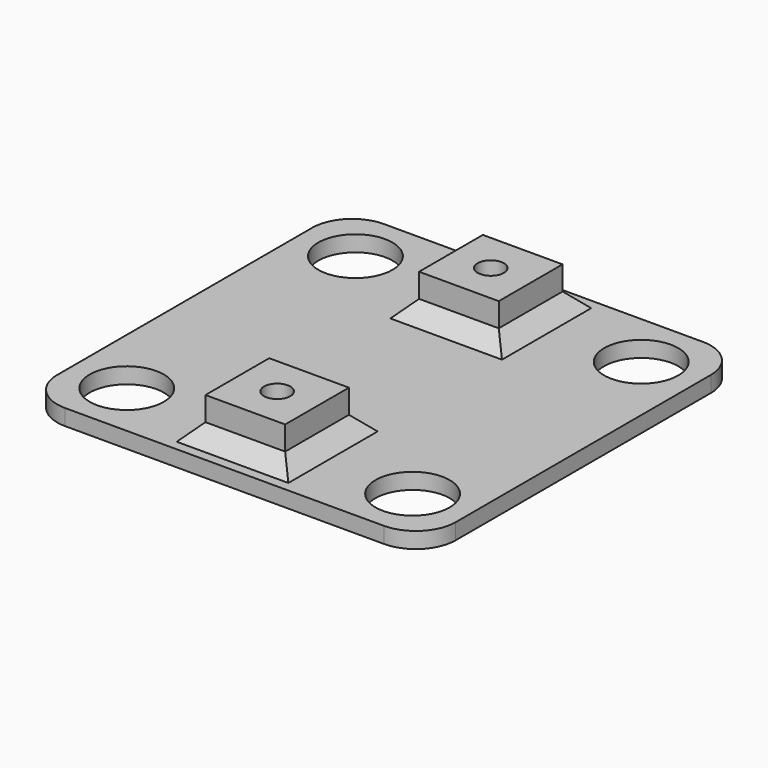
from build123d import *

# Parameters (mm, degrees)
F0_W     = 10
F0_H     = 10
F0_R     = 1.65
F1_DEPTH = 7
F0_R_2   = 4.65
F2_DEPTH = 2
F3_SIZE  = 2


with BuildPart() as f1:
    # F0 (on Top) → F1 (new body)
    with BuildSketch(Plane.XY):
        with Locations((25, -41.75)):
            Rectangle(F0_W, F0_H)
        with Locations((25, -41.75)):
            Circle(F0_R, mode=Mode.SUBTRACT)
    extrude(amount=F1_DEPTH)



with BuildPart() as f1b:
    # F0 (on Top) → F1, piece 2 (new body)
    with BuildSketch(Plane.XY):
        with Locations((25, -8.25)):
            Rectangle(F0_W, F0_H)
        with Locations((25, -8.25)):
            Circle(F0_R, mode=Mode.SUBTRACT)
    extrude(amount=F1_DEPTH)


with BuildPart() as f1_1:
    add(f1.part)

    add(f1b.part)  # F2 merges F1b
    # F0 (on Top) → F2 (join)
    with BuildSketch(Plane.XY):
        with BuildLine():
            Line((45, 0), (5, 0))
            ThreePointArc((5, 0), (1.4644660941, -1.4644660941), (0, -5))
            Line((0, -5), (0, -45))
            ThreePointArc((0, -45), (1.4644660941, -48.5355339059), (5, -50))
            Line((5, -50), (45, -50))
            ThreePointArc((45, -50), (48.5355339059, -48.5355339059), (50, -45))
            Line((50, -45), (50, -5))
            ThreePointArc((50, -5), (48.5355339059, -1.4644660941), (45, 0))
        make_face()
        with Locations((7.0710678119, -42.9289321881)):
            Circle(F0_R_2, mode=Mode.SUBTRACT)
        with Locations((25, -41.75)):
            Rectangle(F0_W, F0_H, mode=Mode.SUBTRACT)
        with Locations((42.9289321881, -42.9289321881)):
            Circle(F0_R_2, mode=Mode.SUBTRACT)
        with Locations((7.0710678119, -7.0710678119)):
            Circle(F0_R_2, mode=Mode.SUBTRACT)
        with Locations((25, -8.25)):
            Rectangle(F0_W, F0_H, mode=Mode.SUBTRACT)
        with Locations((42.9289321881, -7.0710678119)):
            Circle(F0_R_2, mode=Mode.SUBTRACT)
    extrude(amount=F2_DEPTH)

    # F3
    f3_edges = [f1_1.edges().sort_by_distance(p)[0] for p in [
        (25, -46.75, 2),
        (30, -8.25, 2),
        (30, -41.75, 2),
        (25, -13.25, 2),
        (25, -3.25, 2),
        (25, -36.75, 2),
        (20, -8.25, 2),
        (20, -41.75, 2),
    ]]
    chamfer(f3_edges, length=F3_SIZE)


solid = f1_1.part
